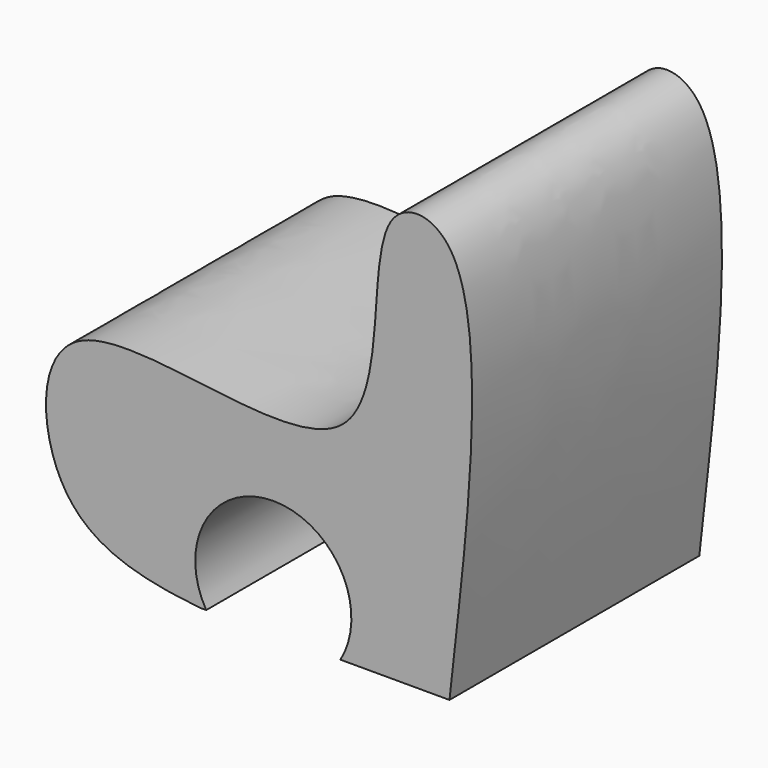
from build123d import *

# Parameters (mm, degrees)
F2_DEPTH = 50
F4_D     = 25


# Not quite as in the source:
# - a feature of the source that left no trace in its solid (it failed there, or was rolled back) is left out
# - the program builds the solid bodies; features that only make, move or delete a surface that nothing else refers to are left out


with BuildPart() as f2:
    # F1 (on Front) → F2 (new body)
    with BuildSketch(Plane.XZ):
        with BuildLine():
            add(Edge.make_bspline(
                [(-39.9705171585, 0), (-51.0732766987, 1.1455419157), (-65.2776511041, 5.7891437868), (-66.4366481756, 43.0274336767), (-5.2696100533, 17.6271931389), (-15.4772339938, 68.279140425), (8.9637191209, 66.9549032244), (2.0169374245, 19.1500262298), (0, 0)],
                knots=[0, 0, 0, 0, 0.1518425407, 0.2910338335, 0.489068508, 0.6625319848, 0.7561455289, 1, 1, 1, 1], degree=3))
            Line((-39.9705171585, 0), (0, 0))
        make_face()
    extrude(amount=F2_DEPTH)

    # F4 (through all)
    with Locations(Plane(origin=(0, 0, 0), x_dir=(1, 0, 0), z_dir=(0, 1, 0))):
        with Locations((-28.2071828842, -6.3905711286)):
            Hole(F4_D / 2)


solid = f2.part
